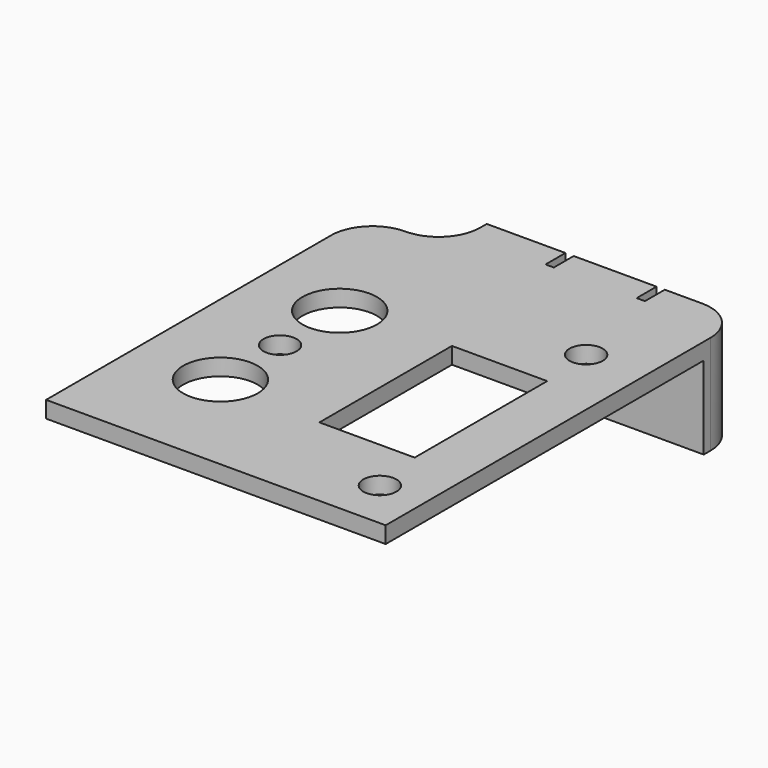
from build123d import *

# Parameters (mm, degrees)
F0_W     = 40
F0_H     = 48
F0_R     = 4.5
F0_R_2   = 2
F0_W_2   = 11.5
F0_H_2   = 20
F1_DEPTH = 2
F2_W     = 31
F2_H     = 12
F3_DEPTH = 6
F4_W     = 1
F4_H     = 12
F5_DEPTH = 3
F6_DEPTH = 1
F7_R     = 4.99999
F8_R     = 5


# Not quite as in the source:
# - a fillet or chamfer is up to 0.001 mm smaller than in the source, because OpenCascade refuses the exact size


with BuildPart() as f1:
    # F0 (on Top) → F1 (new body)
    with BuildSketch(Plane.XY):
        with Locations((20, 24)):
            Rectangle(F0_W, F0_H)
        with Locations((10.25, 13.5)):
            Circle(F0_R, mode=Mode.SUBTRACT)
        with Locations((10.25, 22.5)):
            Circle(F0_R_2, mode=Mode.SUBTRACT)
        with Locations((35.5, 6)):
            Circle(F0_R_2, mode=Mode.SUBTRACT)
        with Locations((28.75, 22.5)):
            Rectangle(F0_W_2, F0_H_2, mode=Mode.SUBTRACT)
        with Locations((10.25, 31.5)):
            Circle(F0_R, mode=Mode.SUBTRACT)
        with Locations((34, 39)):
            Circle(F0_R_2, mode=Mode.SUBTRACT)
    extrude(amount=F1_DEPTH)

    # F2 (on face) → F3 (join)
    with BuildSketch(Plane(origin=(0, 48, 0), x_dir=(-1, 0, 0), z_dir=(0, 1, 0))):
        with Locations((-25.5, -4)):
            Rectangle(F2_W, F2_H)
    extrude(amount=F3_DEPTH)

    # F4 (on face) → F5 (cut)
    with BuildSketch(Plane(origin=(0, 54, 0), x_dir=(-1, 0, 0), z_dir=(0, 1, 0))):
        with Locations((-20, -4)):
            Rectangle(F4_W, F4_H)
        with Locations((-31, -4)):
            Rectangle(F4_W, F4_H)
    extrude(amount=-F5_DEPTH, mode=Mode.SUBTRACT)

    # F6 (add): a face of the model
    f6_faces = [f1.faces().sort_by_distance(p)[0] for p in [
        (40, 24, 1),
    ]]
    extrude(f6_faces, amount=F6_DEPTH)

    # F7 (radius 5 in the source; OpenCascade refuses exactly that, so slightly less here)
    f7_edges = [f1.edges().sort_by_distance(p)[0] for p in [
        (10, 48, 1),
        (0, 48, 1),
    ]]
    fillet(f7_edges, radius=F7_R)

    # F8
    f8_edges = [f1.edges().sort_by_distance(p)[0] for p in [
        (41, 54, -4),
    ]]
    fillet(f8_edges, radius=F8_R)


solid = f1.part
